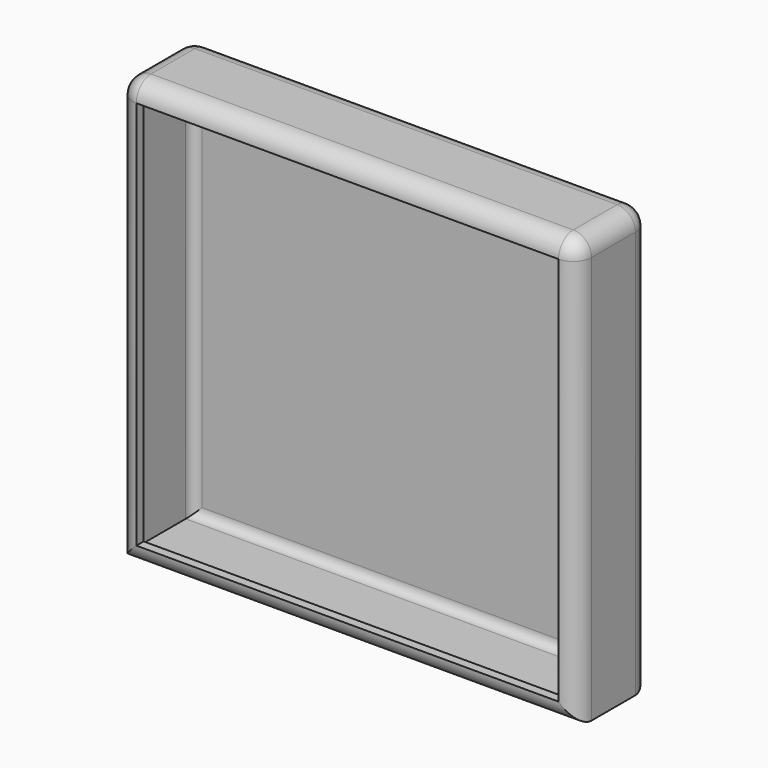
from build123d import *

# Parameters (mm, degrees)
F0_W     = 125.545039773
F0_H     = 116.582095623
F1_DEPTH = 12.5
F2_R     = 5
F3_T     = -2.5


# Not quite as in the source:
# - a shell that OpenCascade refuses in one call is made with other operations: the cavity is built on its own and cut out


with BuildPart() as f1:
    # F0 (on Front) → F1 (new body, symmetric)
    with BuildSketch(Plane.XZ):
        Rectangle(F0_W, F0_H)
    extrude(amount=F1_DEPTH, both=True)

    # F2
    f2_edges = [f1.edges().sort_by_distance(p)[0] for p in [
        (62.77252, 0, 58.291048),
        (0, 12.5, 58.291048),
        (-62.77252, 0, 58.291048),
        (0, -12.5, 58.291048),
        (62.77252, 12.5, 0),
        (0, -12.5, -58.291048),
        (62.77252, -12.5, 0),
        (-62.77252, -12.5, 0),
        (-62.77252, 12.5, 0),
        (0, 12.5, -58.291048),
    ]]
    fillet(f2_edges, radius=F2_R)

    # F3: a shell. OpenCascade refuses it in one call, so the cavity is built on its own and cut out:
    # the body offset inwards by the wall thickness, plus a prism from it out through each open face.
    f3_core = offset(f1.part, amount=F3_T, mode=Mode.PRIVATE)
    f3_exits = [f3_core.faces().sort_by_distance(p)[0] for p in [
        (0, -10, 0),
    ]]
    add(f3_core, mode=Mode.SUBTRACT)
    extrude(f3_exits, amount=-F3_T, mode=Mode.SUBTRACT)


solid = f1.part
